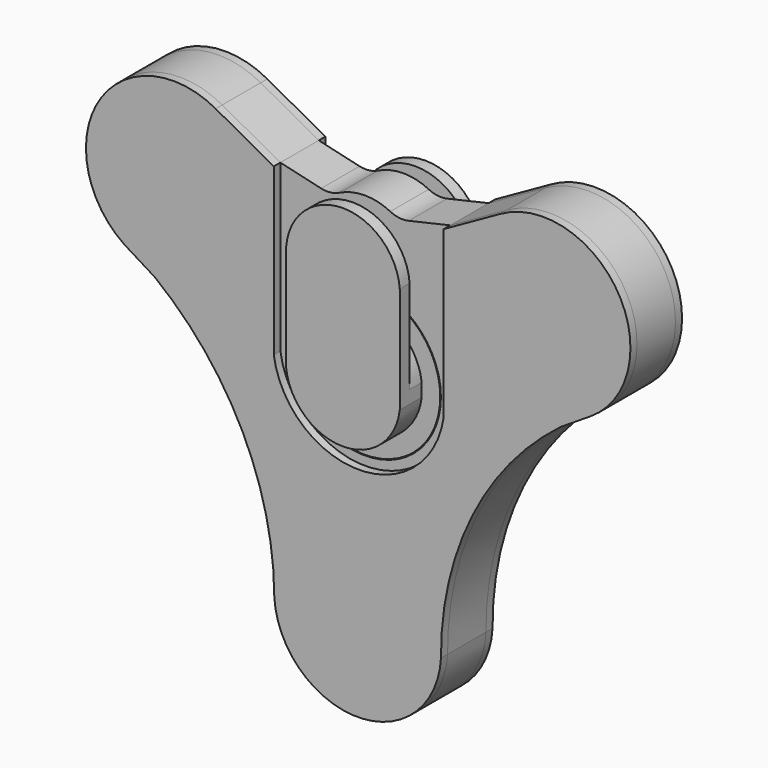
from build123d import *

# Parameters (mm, degrees)
F1_START  = 4.375
F1_DEPTH  = 1.5
F2_R      = 13.875
F3_DEPTH  = 4.375
F5_START  = -4.375
F5_DEPTH  = 1.5
F10_START = 7.125
F10_DEPTH = 2.25
F11_START = -5.5
F11_DEPTH = 2
F12_START = 4.375
F12_DEPTH = 2.75
F13_START = -3.5
F13_DEPTH = 2
F16_START = 0.1
F14_R     = 5.1
F16_DEPTH = 4.275
F17_START = -0.395
F15_R     = 4.14
F17_DEPTH = 3.105
F18_R     = 13.75
F18_R_2   = 4.9375
F19_DEPTH = 4.375
F20_SCALE = 0.8


# Not quite as in the source:
# - a feature names something its author has since deleted; it is built from what else it names


with BuildPart() as f1:
    # F0 (on Front) → F1 (new body)
    with BuildSketch(Plane.XZ.offset(F1_START)):
        with BuildLine():
            Line((25.2868216485, 45.5188639462), (14.9562442675, 39.715051651))
            Line((14.9562442675, 39.715051651), (14.9562442675, 9.5035806298))
            ThreePointArc((14.9562442675, 9.5035806298), (-0.5198442377, -3.9046924703), (-15.995932743, 9.5035806298))
            Line((-15.995932743, 9.5035806298), (-15.995932743, 39.715051651))
            Line((-15.995932743, 39.715051651), (-26.5831723809, 45.5188639462))
            ThreePointArc((-26.5831723809, 45.5188639462), (-47.8560530267, 39.8727264749), (-43.2591997087, 18.3487106115))
            Line((-43.2591997087, 18.3487106115), (-37.7070344985, 14.9252964184))
            ThreePointArc((-37.7070344985, 14.9252964184), (-21.6988985987, -4.6496789904), (-15.8998668194, -29.262913391))
            ThreePointArc((-15.8998668194, -29.262913391), (-0.7185637951, -43.6390577842), (14.4627392292, -29.262913391))
            ThreePointArc((14.4627392292, -29.262913391), (20.148592377, -4.5950626204), (36.2665131688, 14.9252964184))
            Line((36.2665131688, 14.9252964184), (41.6454896331, 18.3487106115))
            ThreePointArc((41.6454896331, 18.3487106115), (46.7179439882, 39.9124542781), (25.2868216485, 45.5188639462))
        make_face()
    extrude(amount=F1_DEPTH)


with BuildPart() as f3:
    # F2 (on Front) → F3 (new body, symmetric)
    with BuildSketch(Plane.XZ):
        with BuildLine():
            ThreePointArc((7.3808994443, 37.9791115091), (5.6737072201, 37.8877583952), (4.0355361424, 38.3768863971))
            ThreePointArc((4.0355361424, 38.3768863971), (-0.5865597778, 39.4647162659), (-5.209378452, 38.3799619045))
            ThreePointArc((-5.209378452, 38.3799619045), (-6.854306785, 37.8911677077), (-8.5676256765, 37.9873309216))
            Line((-8.5676256765, 37.9873309216), (-15.995932743, 39.715051651))
            Line((-15.995932743, 39.715051651), (-26.5831723809, 45.5188639462))
            ThreePointArc((-26.5831723809, 45.5188639462), (-47.8560530267, 39.8727264749), (-43.2591997087, 18.3487106115))
            Line((-43.2591997087, 18.3487106115), (-37.7070344985, 14.9252964184))
            ThreePointArc((-37.7070344985, 14.9252964184), (-21.6988985987, -4.6496789904), (-15.8998668194, -29.262913391))
            ThreePointArc((-15.8998668194, -29.262913391), (-0.7185637951, -43.6390577842), (14.4627392292, -29.262913391))
            ThreePointArc((14.4627392292, -29.262913391), (20.148592377, -4.5950626204), (36.2665131688, 14.9252964184))
            Line((36.2665131688, 14.9252964184), (41.6454896331, 18.3487106115))
            ThreePointArc((41.6454896331, 18.3487106115), (46.7179439882, 39.9124542781), (25.2868216485, 45.5188639462))
            Line((25.2868216485, 45.5188639462), (14.9562442675, 39.715051651))
            Line((14.9562442675, 39.715051651), (7.3808994443, 37.9791115091))
        make_face()
        with Locations((-0.7185637951, -28.4352076707)):
            Circle(F2_R, mode=Mode.SUBTRACT)
        with Locations((-0.6148405476, 11.6066905533)):
            Circle(F2_R, mode=Mode.SUBTRACT)
        with Locations((-34.2546339944, 31.5246824765)):
            Circle(F2_R, mode=Mode.SUBTRACT)
        with Locations((33.1286761467, 31.7305968542)):
            Circle(F2_R, mode=Mode.SUBTRACT)
    extrude(amount=F3_DEPTH, both=True)


with BuildPart() as f5:
    # F4 (on Front) → F5 (new body)
    with BuildSketch(Plane.XZ.offset(F5_START)):
        with BuildLine():
            Line((25.2868216485, 45.5188639462), (14.9562442675, 39.715051651))
            Line((14.9562442675, 39.715051651), (14.9562442675, 9.5035806298))
            ThreePointArc((14.9562442675, 9.5035806298), (-0.5198442377, -3.9046924703), (-15.995932743, 9.5035806298))
            Line((-15.995932743, 9.5035806298), (-15.995932743, 39.715051651))
            Line((-15.995932743, 39.715051651), (-26.5831723809, 45.5188639462))
            ThreePointArc((-26.5831723809, 45.5188639462), (-47.8560530267, 39.8727264749), (-43.2591997087, 18.3487106115))
            Line((-43.2591997087, 18.3487106115), (-37.7070344985, 14.9252964184))
            ThreePointArc((-37.7070344985, 14.9252964184), (-21.6988985987, -4.6496789904), (-15.8998668194, -29.262913391))
            ThreePointArc((-15.8998668194, -29.262913391), (-0.7185637951, -43.6390577842), (14.4627392292, -29.262913391))
            ThreePointArc((14.4627392292, -29.262913391), (20.148592377, -4.5950626204), (36.2665131688, 14.9252964184))
            Line((36.2665131688, 14.9252964184), (41.6454896331, 18.3487106115))
            ThreePointArc((41.6454896331, 18.3487106115), (46.7179439882, 39.9124542781), (25.2868216485, 45.5188639462))
        make_face()
    extrude(amount=-F5_DEPTH)


with BuildPart() as f10:
    # F6 (on Front) → F10 (new body)
    with BuildSketch(Plane.XZ.offset(F10_START)):
        with BuildLine():
            ThreePointArc((9.7599746659, 29.8606865108), (-0.589103438, 39.4640683192), (-10.9381815419, 29.8606865108))
            Line((-10.9381815419, 29.8606865108), (-10.9381815419, 10.4503789917))
            ThreePointArc((-10.9381815419, 10.4503789917), (-0.589103438, 1.2185059392), (9.7599746659, 10.4503789917))
            Line((9.7599746659, 10.4503789917), (9.7599746659, 29.8606865108))
        make_face()
    extrude(amount=F10_DEPTH)

    # F8 (on Front) → F12 (join)
    with BuildSketch(Plane.XZ.offset(F12_START)):
        with BuildLine():
            Line((9.7599746659, 10.4503789917), (9.7599746659, 12.819988866))
            ThreePointArc((9.7599746659, 12.819988866), (-0.589103438, 22.0518619185), (-10.9381815419, 12.819988866))
            Line((-10.9381815419, 12.819988866), (-10.9381815419, 10.4503789917))
            ThreePointArc((-10.9381815419, 10.4503789917), (-0.589103438, 1.2185059392), (9.7599746659, 10.4503789917))
        make_face()
    extrude(amount=F12_DEPTH)

    # F14 (on Front) → F16 (join)
    with BuildSketch(Plane.XZ.offset(F16_START)):
        with Locations((-0.5877316771, 11.6080907404)):
            Circle(F14_R)
    extrude(amount=F16_DEPTH)


with BuildPart() as f11:
    # F7 (on Front) → F11 (new body)
    with BuildSketch(Plane.XZ.offset(F11_START)):
        with BuildLine():
            ThreePointArc((9.7599746659, 29.8606865108), (-0.589103438, 39.4640683192), (-10.9381815419, 29.8606865108))
            Line((-10.9381815419, 29.8606865108), (-10.9381815419, 10.4503789917))
            ThreePointArc((-10.9381815419, 10.4503789917), (-0.589103438, 1.2185059392), (9.7599746659, 10.4503789917))
            Line((9.7599746659, 10.4503789917), (9.7599746659, 29.8606865108))
        make_face()
    extrude(amount=-F11_DEPTH)

    # F9 (on Front) → F13 (join)
    with BuildSketch(Plane.XZ.offset(F13_START)):
        with BuildLine():
            Line((9.7599746659, 10.4503789917), (9.7599746659, 12.819988866))
            ThreePointArc((9.7599746659, 12.819988866), (-0.589103438, 22.0518619185), (-10.9381815419, 12.819988866))
            Line((-10.9381815419, 12.819988866), (-10.9381815419, 10.4503789917))
            ThreePointArc((-10.9381815419, 10.4503789917), (-0.589103438, 1.2185059392), (9.7599746659, 10.4503789917))
        make_face()
    extrude(amount=-F13_DEPTH)

    # F15 (on Front) → F17 (join)
    with BuildSketch(Plane.XZ.offset(F17_START)):
        with Locations((-0.589103438, 11.6351839289)):
            Circle(F15_R)
    extrude(amount=-F17_DEPTH)


with BuildPart() as f19:
    # F18 (on Front) → F19 (new body, symmetric)
    with BuildSketch(Plane.XZ):
        with Locations((-0.6148405476, 11.6066905533)):
            Circle(F18_R)
        with Locations((-0.6148405476, 11.6066905533)):
            Circle(F18_R_2, mode=Mode.SUBTRACT)
    extrude(amount=F19_DEPTH, both=True)


with BuildPart() as f3_1:
    # F20: moved
    add(f3.part.scale(F20_SCALE))


with BuildPart() as f5_1:
    # F20: moved
    add(f5.part.scale(F20_SCALE))


with BuildPart() as f10_1:
    # F20: moved
    add(f10.part.scale(F20_SCALE))


with BuildPart() as f11_1:
    # F20: moved
    add(f11.part.scale(F20_SCALE))


with BuildPart() as f1_1:
    # F20: moved
    add(f1.part.scale(F20_SCALE))


with BuildPart() as f19_1:
    # F20: moved
    add(f19.part.scale(F20_SCALE))


with BuildPart() as f22_1:
    # F22: instance of F10
    add(f10_1.part.mirror(Plane.XZ))


solid = Compound([f3_1.part, f5_1.part, f10_1.part, f1_1.part, f19_1.part, f22_1.part])
